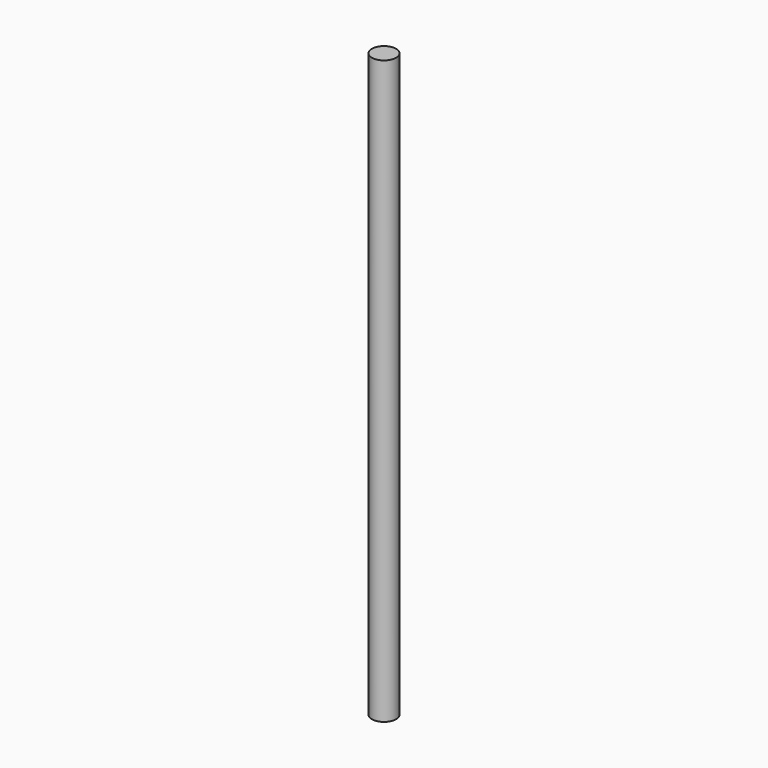
from build123d import *

# Parameters (mm, degrees)
F1_R     = 1.5
F2_DEPTH = 72


with BuildPart() as f2:
    # F1 (on Top) → F2 (new body)
    with BuildSketch(Plane.XY):
        Circle(F1_R)
    extrude(amount=F2_DEPTH)


solid = f2.part
